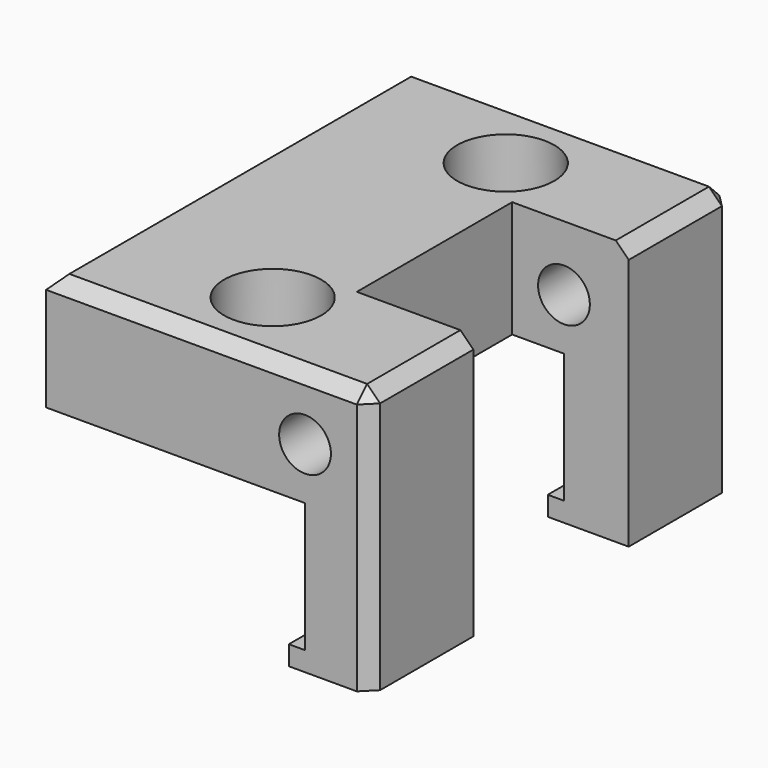
from build123d import *

# Parameters (mm, degrees)
F0_R           = 4
F1_DEPTH       = 35
F3_SIZE        = 2
F2_W           = 18
F2_H           = 41
F4_DEPTH       = 15
F6_D           = 8.4
F6_CBORE_D     = 15
F6_CBORE_DEPTH = 8


# Not quite as in the source:
# - a pattern or mirror of a feature is missing from the dataset's text; its kind, count and spacing are read off the source's solid


with BuildPart() as f1:
    # F0 (on Front) → F1 (new body, symmetric)
    with BuildSketch(Plane.XZ):
        Polygon((-40, 0), (0, 0), (0, -20), (-2.5, -20), (-2.5, -23), (10, -23), (10, 18), (-40, 18), align=None)
        with Locations((0, 8)):
            Circle(F0_R, mode=Mode.SUBTRACT)
    extrude(amount=F1_DEPTH, both=True)

    # F3
    f3_edges = [f1.edges().sort_by_distance(p)[0] for p in [
        (10, 0, 18),
        (10, -35, -2.5),
        (10, 35, -2.5),
        (-15, 35, 18),
        (-15, -35, 18),
        (-40, 0, 18),
    ]]
    chamfer(f3_edges, length=F3_SIZE)

    # F2 (on Front) → F4 (cut, symmetric)
    with BuildSketch(Plane.XZ):
        with Locations((1, -2.5)):
            Rectangle(F2_W, F2_H)
    extrude(amount=F4_DEPTH, both=True, mode=Mode.SUBTRACT)

    # F6 (through all)
    with Locations(Plane.XY.offset(18)):
        with Locations((-15, 22.5)):
            f6 = CounterBoreHole(F6_D / 2, F6_CBORE_D / 2, F6_CBORE_DEPTH)

    # F6_copies: F6 across plane
    add(f6.mirror(Plane(origin=(0, 0, 0), x_dir=(0, 0, -1), z_dir=(0, -1, 0))), mode=Mode.SUBTRACT)


solid = f1.part
